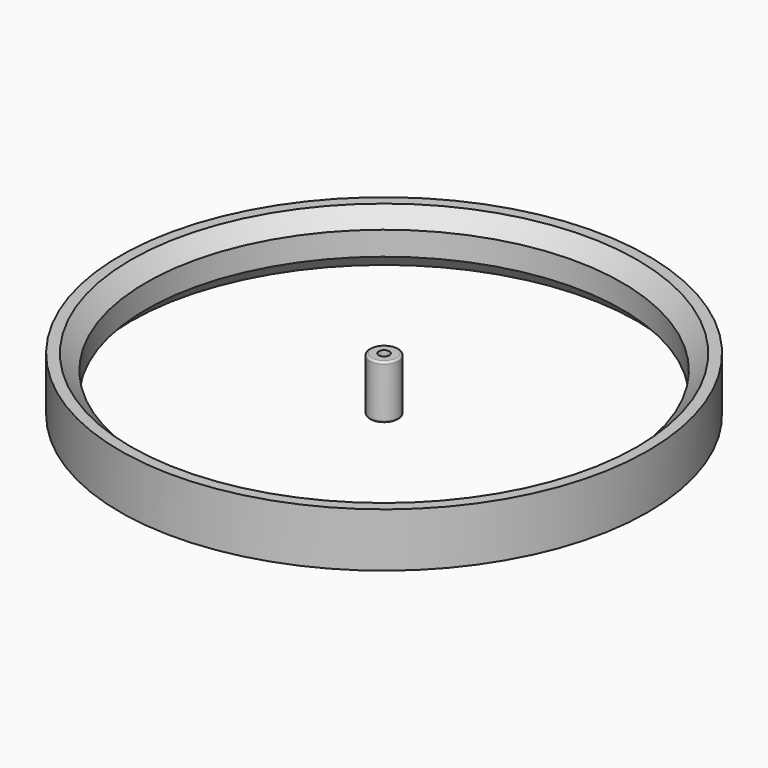
from build123d import *

# Parameters (mm, degrees)
F0_R     = 310.378453622
F1_DEPTH = 31.75
F3_T     = -30.4799746
F2_R     = 17.1053876609
F4_DEPTH = 63.5
F5_R     = 2.54
F9_SIZE  = 17.78
F11_D    = 12.7


# Not quite as in the source:
# - a feature of the source that left no trace in its solid (it failed there, or was rolled back) is left out
# - the program builds the solid bodies; features that only make, move or delete a surface that nothing else refers to are left out


with BuildPart() as f1:
    # F0 (on Top) → F1 (new body, symmetric)
    with BuildSketch(Plane.XY):
        Circle(F0_R)
    extrude(amount=F1_DEPTH, both=True)

    # F3
    f3_openings = [f1.faces().sort_by_distance(p)[0] for p in [
        (0, 0, 31.75),
        (0, 0, -31.75),
    ]]
    offset(amount=F3_T, openings=f3_openings)

    # F9
    f9_edges = [f1.edges().sort_by_distance(p)[0] for p in [
        (-279.898479, 0, -31.75),
        (-279.898479, 0, 31.75),
    ]]
    chamfer(f9_edges, length=F9_SIZE)


with BuildPart() as f4:
    # F2 (on face) → F4 (new body)
    with BuildSketch(Plane.XY.offset(31.75)):
        Circle(F2_R)
    extrude(amount=-F4_DEPTH)

    # F5
    f5_edges = [f4.edges().sort_by_distance(p)[0] for p in [
        (17.105388, 0, 0),
        (-17.105388, 0, 31.75),
        (-17.105388, 0, -31.75),
    ]]
    fillet(f5_edges, radius=F5_R)

    # F11 (through all)
    with Locations(Plane(origin=(0, 0, -31.75), x_dir=(1, 0, 0), z_dir=(0, 0, -1))):
        with Locations((0, 0)):
            Hole(F11_D / 2)


solid = Compound([f1.part, f4.part])
